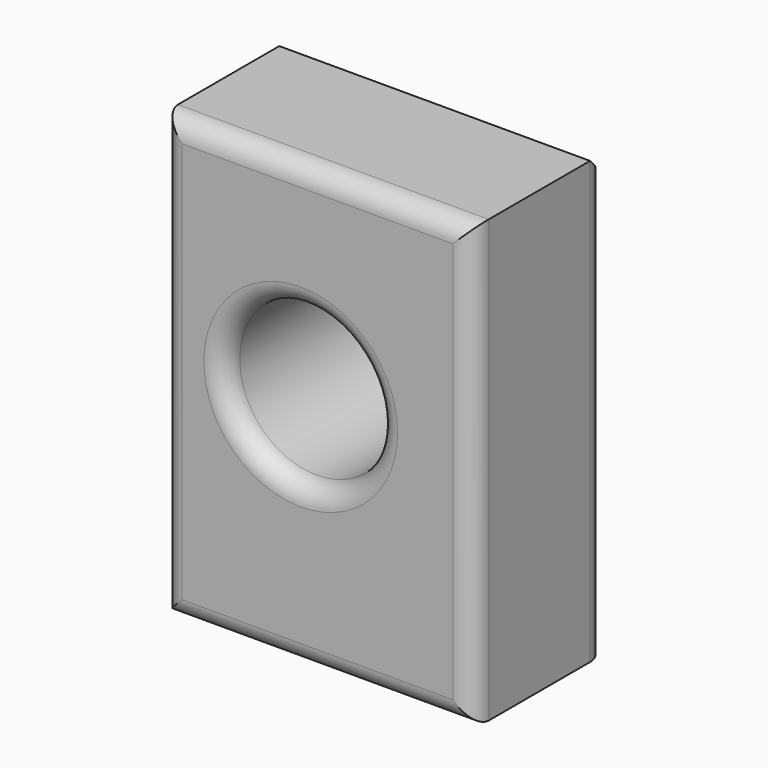
from build123d import *

# Parameters (mm, degrees)
F0_W     = 79.1909694672
F0_H     = 112.4388724566
F0_R     = 19.6004589853
F1_DEPTH = 21.209
F2_R     = 5.08
F3_SIZE  = 5.08
F4_R     = 5.08


# Not quite as in the source:
# - a feature names something its author has since deleted; it is built from what else it names


with BuildPart() as f1:
    # F0 (on Front) → F1 (new body, symmetric)
    with BuildSketch(Plane.XZ):
        with Locations((-183.0625087023, 9.1222152114)):
            Rectangle(F0_W, F0_H)
        with Locations((-187.305867672, 13.2941789925)):
            Circle(F0_R, mode=Mode.SUBTRACT)
    extrude(amount=F1_DEPTH, both=True)

    # F2
    f2_edges = [f1.edges().sort_by_distance(p)[0] for p in [
        (-183.062509, -21.209, 65.341651),
        (-222.657993, -21.209, 9.122215),
        (-183.062509, -21.209, -47.097221),
        (-143.467024, -21.209, 9.122215),
        (-206.906327, -21.209, 13.294179),
    ]]
    fillet(f2_edges, radius=F2_R)

    # F3
    f3_edges = [f1.edges().sort_by_distance(p)[0] for p in [
        (-183.062509, 21.209, 65.341651),
    ]]
    chamfer(f3_edges, length=F3_SIZE)

    # F4
    f4_edges = [f1.edges().sort_by_distance(p)[0] for p in [
        (-143.467024, 21.209, 6.582215),
    ]]
    fillet(f4_edges, radius=F4_R)


solid = f1.part
